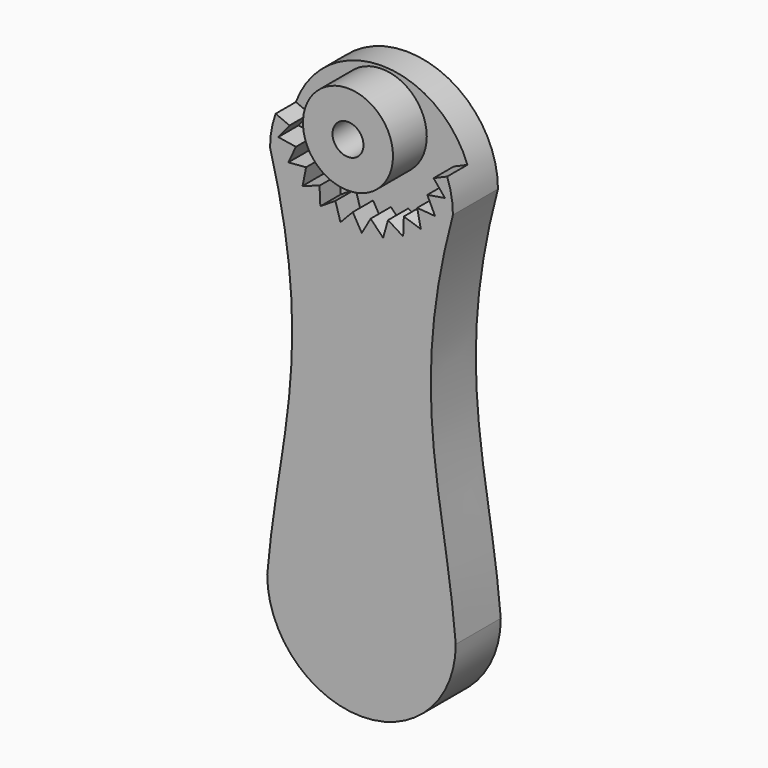
from build123d import *

# Parameters (mm, degrees)
F1_DEPTH = 10.16
F2_R     = 8.128
F2_R_2   = 2.794
F3_DEPTH = 3.048
F4_DEPTH = 50.8
F5_R     = 8.128
F6_DEPTH = 4.572
F7_R     = 5.08
F7_R_2   = 2.794
F8_DEPTH = 5.08


with BuildPart() as f1:
    # F0 (on Front) → F1 (new body)
    with BuildSketch(Plane.XZ):
        with BuildLine():
            add(Edge.make_bspline(
                [(16.51, 16.2022389048), (8.1950903917, -14.7107664531), (15.1309384414, -29.2677398155), (17.018, -51.8697610952)],
                knots=[0, 0, 0, 0, 68.073895496, 68.073895496, 68.073895496, 68.073895496], degree=3))
            ThreePointArc((16.51, 16.2022389048), (0, 32.7122389048), (-16.51, 16.2022389048))
            add(Edge.make_bspline(
                [(-16.51, 16.2022389048), (-8.1950903917, -14.7107664531), (-15.1309384414, -29.2677398155), (-17.018, -51.8697610952)],
                knots=[0, 0, 0, 0, 68.073895496, 68.073895496, 68.073895496, 68.073895496], degree=3))
            ThreePointArc((-17.018, -51.8697610952), (0, -68.8877610952), (17.018, -51.8697610952))
        make_face()
    extrude(amount=F1_DEPTH)

    # F2 (on face) → F3 (join)
    with BuildSketch(Plane.XZ.offset(10.16)):
        with Locations((0, 24.0762389048)):
            Circle(F2_R)
        with Locations((0, 24.0762389048)):
            Circle(F2_R_2, mode=Mode.SUBTRACT)
    extrude(amount=F3_DEPTH)

    # F4 (cut, symmetric): a face of the model
    f4_faces = [f1.faces().sort_by_distance(p)[0] for p in [
        (0, -10.16, 24.0762389048),
    ]]
    extrude(f4_faces, amount=F4_DEPTH, both=True, mode=Mode.SUBTRACT)

    # F5 (on face) → F6 (cut)
    with BuildSketch(Plane.XZ.offset(10.16)):
        with BuildLine():
            ThreePointArc((15.469928865, 21.9695087018), (-0.0442530739, 32.7121795972), (-15.5006234178, 21.8864955545))
            Line((-15.5006234178, 21.8864955545), (-12.9936152173, 20.8281131752))
            Line((-12.9936152173, 20.8281131752), (-15.0273981388, 18.3203464733))
            Line((-15.0273981388, 18.3203464733), (-11.8387170074, 17.8129221485))
            Line((-11.8387170074, 17.8129221485), (-13.2132540393, 14.8913104783))
            Line((-13.2132540393, 14.8913104783), (-9.995795597, 15.1617323254))
            Line((-9.995795597, 15.1617323254), (-10.6312036432, 11.9960691377))
            Line((-10.6312036432, 11.9960691377), (-7.5719548797, 13.0286212217))
            Line((-7.5719548797, 13.0286212217), (-7.4313063342, 9.8028833542))
            Line((-7.4313063342, 9.8028833542), (-4.7080596678, 11.5375575014))
            Line((-4.7080596678, 11.5375575014), (-3.7995285128, 8.4392131139))
            Line((-3.7995285128, 8.4392131139), (-1.570549141, 10.7751963679))
            Line((-1.570549141, 10.7751963679), (0.0530640951, 7.9843099742))
            Line((0.0530640951, 7.9843099742), (1.6582359931, 10.7858434794))
            Line((1.6582359931, 10.7858434794), (3.9025728106, 8.4646112522))
            Line((3.9025728106, 8.4646112522), (4.7906504787, 11.5688800644))
            Line((4.7906504787, 11.5688800644), (7.5252781797, 9.8522035834))
            Line((7.5252781797, 9.8522035834), (7.6446497718, 13.0787988828))
            Line((7.6446497718, 13.0787988828), (10.7106417342, 12.0664451452))
            Line((10.7106417342, 12.0664451452), (10.0543698074, 15.2278489412))
            Line((10.0543698074, 15.2278489412), (13.2735417227, 14.9786522665))
            Line((13.2735417227, 14.9786522665), (11.8797664159, 17.8911352617))
            Line((11.8797664159, 17.8911352617), (15.0650317137, 18.4195780548))
            Line((15.0650317137, 18.4195780548), (13.0147541814, 20.913877324))
            Line((13.0147541814, 20.913877324), (15.469928865, 21.9695087018))
        make_face()
        with BuildLine():
            Line((-11.7664292563, 17.8014187834), (-11.8387170074, 17.8129221485))
            Line((-11.8387170074, 17.8129221485), (-11.8075561021, 17.8791554056))
            ThreePointArc((-11.8075561021, 17.8791554056), (-11.7870567643, 17.84025319), (-11.7664292563, 17.8014187834))
        make_face(mode=Mode.SUBTRACT)
        with BuildLine():
            Line((-9.9228554611, 15.1678628183), (-9.995795597, 15.1617323254))
            Line((-9.995795597, 15.1617323254), (-9.9813908269, 15.2334982572))
            ThreePointArc((-9.9813908269, 15.2334982572), (-9.952177253, 15.2006322819), (-9.9228554611, 15.1678628183))
        make_face(mode=Mode.SUBTRACT)
        with BuildLine():
            Line((-12.9261809524, 20.7996444858), (-12.9936152173, 20.8281131752))
            Line((-12.9936152173, 20.8281131752), (-12.9475091354, 20.8849645215))
            ThreePointArc((-12.9475091354, 20.8849645215), (-12.9369153807, 20.842286921), (-12.9261809524, 20.7996444858))
        make_face(mode=Mode.SUBTRACT)
        with BuildLine():
            Line((-7.5026013746, 13.0520292908), (-7.5719548797, 13.0286212217))
            Line((-7.5719548797, 13.0286212217), (-7.5751433977, 13.1017490531))
            ThreePointArc((-7.5751433977, 13.1017490531), (-7.5389133745, 13.0768293692), (-7.5026013746, 13.0520292908))
        make_face(mode=Mode.SUBTRACT)
        with BuildLine():
            Line((-4.646323367, 11.5768827546), (-4.7080596678, 11.5375575014))
            Line((-4.7080596678, 11.5375575014), (-4.7286561687, 11.6077973086))
            ThreePointArc((-4.7286561687, 11.6077973086), (-4.6875152535, 11.5922721575), (-4.646323367, 11.5768827546))
        make_face(mode=Mode.SUBTRACT)
        with BuildLine():
            Line((-1.5200179341, 10.8281533646), (-1.570549141, 10.7751963679))
            Line((-1.570549141, 10.7751963679), (-1.6073566312, 10.8384660687))
            ThreePointArc((-1.6073566312, 10.8384660687), (-1.5636957843, 10.8332377157), (-1.5200179341, 10.8281533646))
        make_face(mode=Mode.SUBTRACT)
        with BuildLine():
            Line((1.6946254161, 10.8493545514), (1.6582359931, 10.7858434794))
            Line((1.6582359931, 10.7858434794), (1.6073566312, 10.8384660687))
            ThreePointArc((1.6073566312, 10.8384660687), (1.651, 10.8438383667), (1.6946254161, 10.8493545514))
        make_face(mode=Mode.SUBTRACT)
        with BuildLine():
            Line((4.8107832969, 11.639254179), (4.7906504787, 11.5688800644))
            Line((4.7906504787, 11.5688800644), (4.7286561687, 11.6077973086))
            ThreePointArc((4.7286561687, 11.6077973086), (4.7697456655, 11.6234580392), (4.8107832969, 11.639254179))
        make_face(mode=Mode.SUBTRACT)
        with BuildLine():
            Line((7.6473559389, 13.1519461522), (7.6446497718, 13.0787988828))
            Line((7.6446497718, 13.0787988828), (7.5751433977, 13.1017490531))
            ThreePointArc((7.5751433977, 13.1017490531), (7.6112910502, 13.1267880715), (7.6473559389, 13.1519461522))
        make_face(mode=Mode.SUBTRACT)
        with Locations((0, 24.0762389048)):
            Circle(F5_R, mode=Mode.SUBTRACT)
        with BuildLine():
            Line((11.8481693767, 17.9571615707), (11.8797664159, 17.8911352617))
            Line((11.8797664159, 17.8911352617), (11.8075561021, 17.8791554056))
            ThreePointArc((11.8075561021, 17.8791554056), (11.8279270467, 17.9181250071), (11.8481693767, 17.9571615707))
        make_face(mode=Mode.SUBTRACT)
        with BuildLine():
            Line((12.9682741648, 20.9704233621), (13.0147541814, 20.913877324))
            Line((13.0147541814, 20.913877324), (12.9475091354, 20.8849645215))
            ThreePointArc((12.9475091354, 20.8849645215), (12.9579621013, 20.9276768234), (12.9682741648, 20.9704233621))
        make_face(mode=Mode.SUBTRACT)
        with BuildLine():
            Line((-12.9475091354, 20.8849645215), (-12.9936152173, 20.8281131752))
            Line((-12.9936152173, 20.8281131752), (-12.9261809524, 20.7996444858))
            ThreePointArc((-12.9261809524, 20.7996444858), (-12.9369153807, 20.842286921), (-12.9475091354, 20.8849645215))
        make_face()
        with BuildLine():
            Line((-11.8075561021, 17.8791554056), (-11.8387170074, 17.8129221485))
            Line((-11.8387170074, 17.8129221485), (-11.7664292563, 17.8014187834))
            ThreePointArc((-11.7664292563, 17.8014187834), (-11.7870567643, 17.84025319), (-11.8075561021, 17.8791554056))
        make_face()
        with BuildLine():
            Line((-9.9813908269, 15.2334982572), (-9.995795597, 15.1617323254))
            Line((-9.995795597, 15.1617323254), (-9.9228554611, 15.1678628183))
            ThreePointArc((-9.9228554611, 15.1678628183), (-9.952177253, 15.2006322819), (-9.9813908269, 15.2334982572))
        make_face()
        with BuildLine():
            Line((-7.5751433977, 13.1017490531), (-7.5719548797, 13.0286212217))
            Line((-7.5719548797, 13.0286212217), (-7.5026013746, 13.0520292908))
            ThreePointArc((-7.5026013746, 13.0520292908), (-7.5389133745, 13.0768293692), (-7.5751433977, 13.1017490531))
        make_face()
        with BuildLine():
            Line((-4.7286561687, 11.6077973086), (-4.7080596678, 11.5375575014))
            Line((-4.7080596678, 11.5375575014), (-4.646323367, 11.5768827546))
            ThreePointArc((-4.646323367, 11.5768827546), (-4.6875152535, 11.5922721575), (-4.7286561687, 11.6077973086))
        make_face()
        with BuildLine():
            Line((-1.6073566312, 10.8384660687), (-1.570549141, 10.7751963679))
            Line((-1.570549141, 10.7751963679), (-1.5200179341, 10.8281533646))
            ThreePointArc((-1.5200179341, 10.8281533646), (-1.5636957843, 10.8332377157), (-1.6073566312, 10.8384660687))
        make_face()
        with BuildLine():
            Line((1.6073566312, 10.8384660687), (1.6582359931, 10.7858434794))
            Line((1.6582359931, 10.7858434794), (1.6946254161, 10.8493545514))
            ThreePointArc((1.6946254161, 10.8493545514), (1.651, 10.8438383667), (1.6073566312, 10.8384660687))
        make_face()
        with BuildLine():
            Line((4.7286561687, 11.6077973086), (4.7906504787, 11.5688800644))
            Line((4.7906504787, 11.5688800644), (4.8107832969, 11.639254179))
            ThreePointArc((4.8107832969, 11.639254179), (4.7697456655, 11.6234580392), (4.7286561687, 11.6077973086))
        make_face()
        with BuildLine():
            Line((7.5751433977, 13.1017490531), (7.6446497718, 13.0787988828))
            Line((7.6446497718, 13.0787988828), (7.6473559389, 13.1519461522))
            ThreePointArc((7.6473559389, 13.1519461522), (7.6112910502, 13.1267880715), (7.5751433977, 13.1017490531))
        make_face()
        with BuildLine():
            Line((11.8075561021, 17.8791554056), (11.8797664159, 17.8911352617))
            Line((11.8797664159, 17.8911352617), (11.8481693767, 17.9571615707))
            ThreePointArc((11.8481693767, 17.9571615707), (11.8279270467, 17.9181250071), (11.8075561021, 17.8791554056))
        make_face()
        with BuildLine():
            Line((12.9475091354, 20.8849645215), (13.0147541814, 20.913877324))
            Line((13.0147541814, 20.913877324), (12.9682741648, 20.9704233621))
            ThreePointArc((12.9682741648, 20.9704233621), (12.9579621013, 20.9276768234), (12.9475091354, 20.8849645215))
        make_face()
    extrude(amount=-F6_DEPTH, mode=Mode.SUBTRACT)

    # F7 (on face) → F8 (cut)
    with BuildSketch(Plane(origin=(0, 0, 0), x_dir=(-1, 0, 0), z_dir=(0, 1, 0))):
        with Locations((0, 24.0762389048)):
            Circle(F7_R)
        with Locations((0, 24.0762389048)):
            Circle(F7_R_2, mode=Mode.SUBTRACT)
        with Locations((0, 24.0762389048)):
            Circle(F7_R_2)
    extrude(amount=-F8_DEPTH, mode=Mode.SUBTRACT)


solid = f1.part
